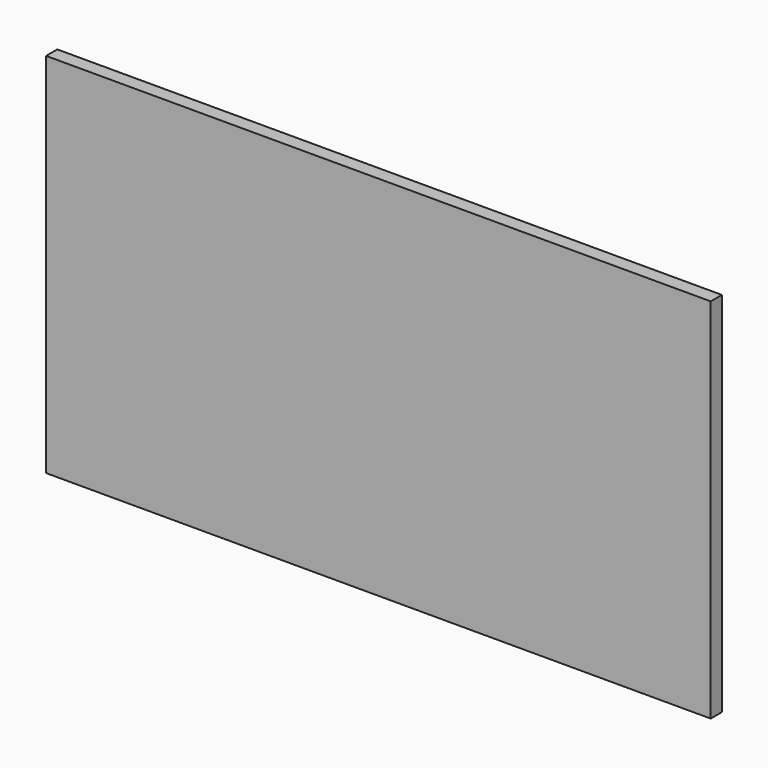
from build123d import *

# Parameters (mm, degrees)
F0_W     = 48260
F0_H     = 26670
F0_W_2   = 32512
F0_H_2   = 10922
F0_W_3   = 30988
F0_H_3   = 9398
F0_R     = 4064
F1_DEPTH = 1016
F2_DEPTH = 1270
F3_DEPTH = 1905
F4_R     = 508
F6_DEPTH = 25


with BuildPart() as f1:
    # F0 (on Front) → F1 (new body)
    with BuildSketch(Plane.XZ):
        Rectangle(F0_W, F0_H)
        Rectangle(F0_W_2, F0_H_2, mode=Mode.SUBTRACT)
        Rectangle(F0_W_2, F0_H_2)
        Rectangle(F0_W_3, F0_H_3, mode=Mode.SUBTRACT)
        Rectangle(F0_W_3, F0_H_3)
        with Locations((8890, 0)):
            Circle(F0_R, mode=Mode.SUBTRACT)
        with Locations((8890, 0)):
            Circle(F0_R)
    extrude(amount=F1_DEPTH)

    # F0 (on Front) → F2 (join)
    with BuildSketch(Plane.XZ):
        Rectangle(F0_W_2, F0_H_2)
        Rectangle(F0_W_3, F0_H_3, mode=Mode.SUBTRACT)
        Rectangle(F0_W_3, F0_H_3)
        with Locations((8890, 0)):
            Circle(F0_R, mode=Mode.SUBTRACT)
    extrude(amount=-F2_DEPTH)

    # F0 (on Front) → F3 (join)
    with BuildSketch(Plane.XZ):
        with Locations((8890, 0)):
            Circle(F0_R)
    extrude(amount=-F3_DEPTH)

    # F4
    f4_edges = [f1.edges().sort_by_distance(p)[0] for p in [
        (16256, 635, -5461),
        (16256, 635, 5461),
        (-16256, 635, -5461),
        (-16256, 635, 5461),
    ]]
    fillet(f4_edges, radius=F4_R)

    # F5 (on face) → F6 (cut)
    with BuildSketch(Plane(origin=(0, 1270, 0), x_dir=(-1, 0, 0), z_dir=(0, 1, 0))):
        with BuildLine():
            Line((8890, 4699), (-8890, 4699))
            add(Edge.make_bspline(
                [(-15494, 0), (-15494, 2701.7158539631), (-11699.5907432682, 4699), (-8890, 4699)],
                knots=[0, 0, 0, 0, 8105.1475618893, 8105.1475618893, 8105.1475618893, 8105.1475618893], degree=3))
            add(Edge.make_bspline(
                [(-15494, 0), (-15494, -2701.7158539631), (-11699.5907432682, -4699), (-8890, -4699)],
                knots=[0, 0, 0, 0, 8105.1475618893, 8105.1475618893, 8105.1475618893, 8105.1475618893], degree=3))
            Line((-8890, -4699), (8890, -4699))
            add(Edge.make_bspline(
                [(15494, 0), (15494, -2701.7158539631), (11699.5907432682, -4699), (8890, -4699)],
                knots=[0, 0, 0, 0, 8105.1475618893, 8105.1475618893, 8105.1475618893, 8105.1475618893], degree=3))
            add(Edge.make_bspline(
                [(15494, 0), (15494, 2701.7158539631), (11699.5907432682, 4699), (8890, 4699)],
                knots=[0, 0, 0, 0, 8105.1475618893, 8105.1475618893, 8105.1475618893, 8105.1475618893], degree=3))
        make_face()
        with BuildLine():
            Line((-8890, 4572), (8890, 4572))
            ThreePointArc((8890, 4572), (13462, 0), (8890, -4572))
            Line((8890, -4572), (-8890, -4572))
            ThreePointArc((-8890, -4572), (-13462, 0), (-8890, 4572))
        make_face(mode=Mode.SUBTRACT)
    extrude(amount=-F6_DEPTH, mode=Mode.SUBTRACT)


solid = f1.part
